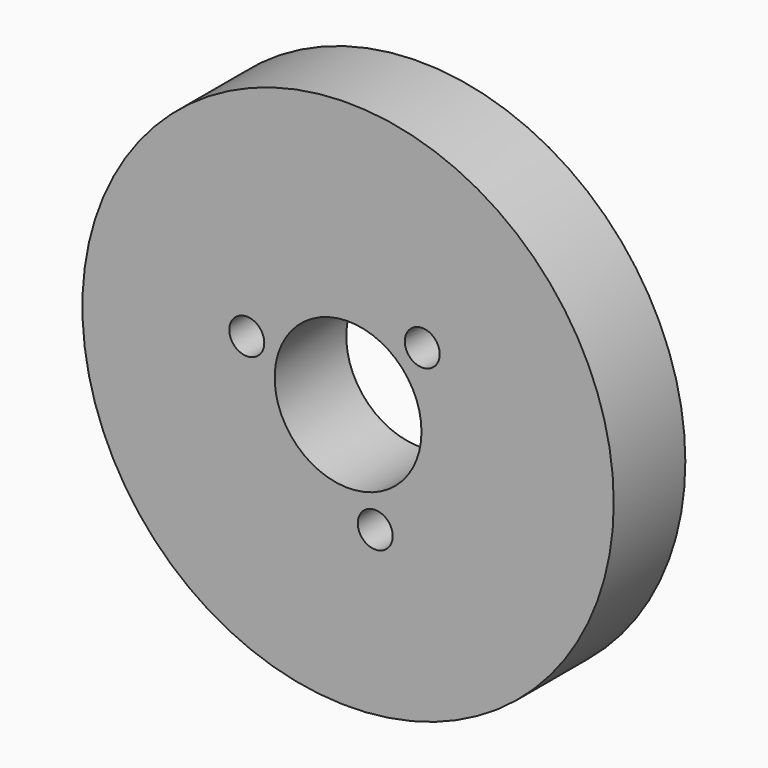
from build123d import *

# Parameters (mm, degrees)
F0_R            = 19
F1_DEPTH        = 6.4
F2_R            = 1.25
F3_DEPTH        = 25.4
F3_COPIES_COUNT = 3
F4_R            = 5.25
F5_DEPTH        = 6.401


# Not quite as in the source:
# - a pattern or mirror of a feature is missing from the dataset's text; its kind, count and spacing are read off the source's solid


with BuildPart() as f1:
    # F0 (on Front) → F1 (new body)
    with BuildSketch(Plane.XZ):
        Circle(F0_R)
    extrude(amount=F1_DEPTH)

    # F2 (on Front) → F3 (cut)
    with BuildSketch(Plane.XZ):
        with Locations((5.3033008589, 5.3033008589)):
            Circle(F2_R)
    f3 = extrude(amount=F3_DEPTH, mode=Mode.SUBTRACT)

    # F3_copies: F3 ×3 about axis
    f3_copies_axis = Axis((0, 0, 0), (0, 1, 0))
    for i in range(1, F3_COPIES_COUNT):
        add(f3.rotate(f3_copies_axis, i * 360 / F3_COPIES_COUNT), mode=Mode.SUBTRACT)

    # F4 (on Front) → F5 (cut, through all)
    with BuildSketch(Plane.XZ):
        Circle(F4_R)
    extrude(amount=F5_DEPTH, mode=Mode.SUBTRACT)


solid = f1.part
